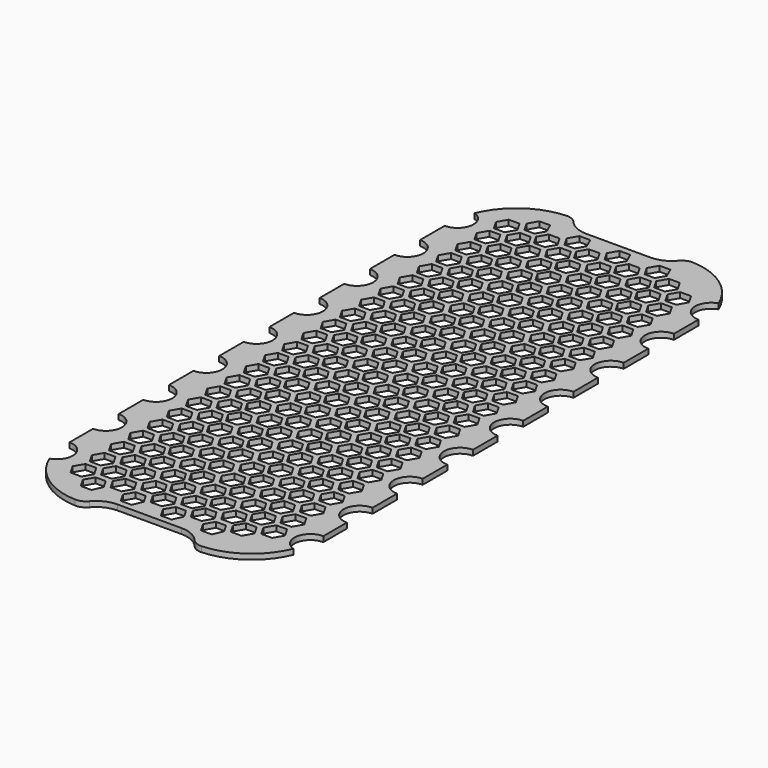
from build123d import *

# Parameters (mm, degrees)
F0_W        = 95
F0_H        = 230
F1_DEPTH    = 2
F2_R        = 25
F3_R        = 6
F3_W        = 41.7297072709
F3_H        = 10
F4_DEPTH    = 10
F5_T1_DEPTH = 2
F6_R        = 5
F8_DEPTH    = 10


# Not quite as in the source:
# - a fillet or chamfer that OpenCascade refuses, or shapes differently, is made with other operations: its cross-section is extruded or revolved along the edge and cut away or added


with BuildPart() as f1:
    # F0 (on Top) → F1 (new body)
    with BuildSketch(Plane.XY):
        Rectangle(F0_W, F0_H)
    extrude(amount=F1_DEPTH)

    # F2
    f2_edges = [f1.edges().sort_by_distance(p)[0] for p in [
        (-47.5, -115, 1),
        (-47.5, 115, 1),
        (47.5, 115, 1),
        (47.5, -115, 1),
    ]]
    fillet(f2_edges, radius=F2_R)

    # F3 (on Top) → F4 (cut)
    with BuildSketch(Plane.XY):
        with Locations((-47.4763996899, 93.75)):
            Circle(F3_R)
        with Locations((47.4763996899, 93.75)):
            Circle(F3_R)
        with Locations((-47.4763996899, -93.75)):
            Circle(F3_R)
        with Locations((47.4763996899, -93.75)):
            Circle(F3_R)
        with Locations((-47.4763996899, 70.25)):
            Circle(F3_R)
        with Locations((-47.4763996899, 46.75)):
            Circle(F3_R)
        with Locations((-47.4763996899, 23.25)):
            Circle(F3_R)
        with Locations((-47.4763996899, -0.25)):
            Circle(F3_R)
        with Locations((-47.4763996899, -23.75)):
            Circle(F3_R)
        with Locations((-47.4763996899, -47.25)):
            Circle(F3_R)
        with Locations((47.4763996899, 70.25)):
            Circle(F3_R)
        with Locations((47.4763996899, 46.75)):
            Circle(F3_R)
        with Locations((47.4763996899, 23.25)):
            Circle(F3_R)
        with Locations((47.4763996899, -0.25)):
            Circle(F3_R)
        with Locations((47.4763996899, -23.75)):
            Circle(F3_R)
        with Locations((47.4763996899, -47.25)):
            Circle(F3_R)
        with Locations((47.4763996899, -70.75)):
            Circle(F3_R)
        with Locations((-47.4763996899, -70.75)):
            Circle(F3_R)
        with Locations((0, -114.6645247936)):
            Rectangle(F3_W, F3_H)
        with Locations((0, 114.6645247936)):
            Rectangle(F3_W, F3_H)
    extrude(amount=F4_DEPTH, mode=Mode.SUBTRACT)

    # F5: fillet of radius 10 on 4 edges, made by hand

    # F5_s2 → F5_t1 (join)
    with BuildSketch(Plane.XY):
        with BuildLine():
            ThreePointArc((-12.0193910444, -109.6645247936), (-17.1844056651, -111.1016617229), (-20.8648536354, -115))
            Line((-20.8648536354, -115), (-20.8648536354, -109.6645247936))
            Line((-20.8648536354, -109.6645247936), (-12.0193910444, -109.6645247936))
        make_face()
        with BuildLine():
            ThreePointArc((20.8648536354, -115), (17.1844056651, -111.1016617229), (12.0193910444, -109.6645247936))
            Line((12.0193910444, -109.6645247936), (20.8648536354, -109.6645247936))
            Line((20.8648536354, -109.6645247936), (20.8648536354, -115))
        make_face()
        with BuildLine():
            ThreePointArc((-20.8648536354, 115), (-17.1844056651, 111.1016617229), (-12.0193910444, 109.6645247936))
            Line((-12.0193910444, 109.6645247936), (-20.8648536354, 109.6645247936))
            Line((-20.8648536354, 109.6645247936), (-20.8648536354, 115))
        make_face()
        with BuildLine():
            ThreePointArc((12.0193910444, 109.6645247936), (17.1844056651, 111.1016617229), (20.8648536354, 115))
            Line((20.8648536354, 115), (20.8648536354, 109.6645247936))
            Line((20.8648536354, 109.6645247936), (12.0193910444, 109.6645247936))
        make_face()
    extrude(amount=F5_T1_DEPTH)

    # F6
    f6_edges = [f1.edges().sort_by_distance(p)[0] for p in [
        (-20.864854, 115, 1),
        (20.864854, 115, 1),
        (-20.864854, -115, 1),
        (20.864854, -115, 1),
    ]]
    fillet(f6_edges, radius=F6_R)

    # F7 (on Top) → F8 (cut)
    with BuildSketch(Plane.XY):
        Polygon((32.4792740578, -91), (30.4585481157, -94.5), (32.4792740578, -98), (36.5207259422, -98), (38.5414518843, -94.5), (36.5207259422, -91), align=None)
        Polygon((32.4725603018, -82.003884784), (30.4585555593, -85.5077566753), (32.4859952575, -89.0038718913), (36.5274396982, -88.996115216), (38.5414444407, -85.4922433247), (36.5140047425, -81.9961281087), align=None)
        Polygon((32.4792740578, -80), (36.5207259422, -80), (38.5414518843, -76.5), (36.5207259422, -73), (32.4792740578, -73), (30.4585481157, -76.5), align=None)
        Polygon((30.4585555593, -67.5077566753), (32.4859952575, -71.0038718913), (36.5274396982, -70.996115216), (38.5414444407, -67.4922433247), (36.5140047425, -63.9961281087), (32.4725603018, -64.003884784), align=None)
        Polygon((32.4792740578, -62), (36.5207259422, -62), (38.5414518843, -58.5), (36.5207259422, -55), (32.4792740578, -55), (30.4585481157, -58.5), align=None)
        Polygon((30.4585555593, -49.5077566753), (32.4859952575, -53.0038718913), (36.5274396982, -52.996115216), (38.5414444407, -49.4922433247), (36.5140047425, -45.9961281087), (32.4725603018, -46.003884784), align=None)
        Polygon((32.4792740578, -44), (36.5207259422, -44), (38.5414518843, -40.5), (36.5207259422, -37), (32.4792740578, -37), (30.4585481157, -40.5), align=None)
        Polygon((30.4585555593, -31.5077566753), (32.4859952575, -35.0038718913), (36.5274396982, -34.996115216), (38.5414444407, -31.4922433247), (36.5140047425, -27.9961281087), (32.4725603018, -28.003884784), align=None)
        Polygon((32.4792740578, -26), (36.5207259422, -26), (38.5414518843, -22.5), (36.5207259422, -19), (32.4792740578, -19), (30.4585481157, -22.5), align=None)
        Polygon((30.4585555593, -13.5077566753), (32.4859952575, -17.0038718913), (36.5274396982, -16.996115216), (38.5414444407, -13.4922433247), (36.5140047425, -9.9961281087), (32.4725603018, -10.003884784), align=None)
        Polygon((32.4792740578, -8), (36.5207259422, -8), (38.5414518843, -4.5), (36.5207259422, -1), (32.4792740578, -1), (30.4585481157, -4.5), align=None)
        Polygon((30.4585555593, 4.4922433247), (32.4859952575, 0.9961281087), (36.5274396982, 1.003884784), (38.5414444407, 4.5077566753), (36.5140047425, 8.0038718913), (32.4725603018, 7.996115216), align=None)
        Polygon((32.4792740578, 10), (36.5207259422, 10), (38.5414518843, 13.5), (36.5207259422, 17), (32.4792740578, 17), (30.4585481157, 13.5), align=None)
        Polygon((30.4585555593, 22.4922433247), (32.4859952575, 18.9961281087), (36.5274396982, 19.003884784), (38.5414444407, 22.5077566753), (36.5140047425, 26.0038718913), (32.4725603018, 25.996115216), align=None)
        Polygon((32.4792740578, 28), (36.5207259422, 28), (38.5414518843, 31.5), (36.5207259422, 35), (32.4792740578, 35), (30.4585481157, 31.5), align=None)
        Polygon((30.4585555593, 40.4922433247), (32.4859952575, 36.9961281087), (36.5274396982, 37.003884784), (38.5414444407, 40.5077566753), (36.5140047425, 44.0038718913), (32.4725603018, 43.996115216), align=None)
        Polygon((32.4792740578, 46), (36.5207259422, 46), (38.5414518843, 49.5), (36.5207259422, 53), (32.4792740578, 53), (30.4585481157, 49.5), align=None)
        Polygon((30.4585555593, 58.4922433247), (32.4859952575, 54.9961281087), (36.5274396982, 55.003884784), (38.5414444407, 58.5077566753), (36.5140047425, 62.0038718913), (32.4725603018, 61.996115216), align=None)
        Polygon((32.4792740578, 64), (36.5207259422, 64), (38.5414518843, 67.5), (36.5207259422, 71), (32.4792740578, 71), (30.4585481157, 67.5), align=None)
        Polygon((30.4585555593, 76.4922433247), (32.4859952575, 72.9961281087), (36.5274396982, 73.003884784), (38.5414444407, 76.5077566753), (36.5140047425, 80.0038718913), (32.4725603018, 79.996115216), align=None)
        Polygon((32.4792740578, 82), (36.5207259422, 82), (38.5414518843, 85.5), (36.5207259422, 89), (32.4792740578, 89), (30.4585481157, 85.5), align=None)
        Polygon((30.4585555593, 94.4922433247), (32.4859952575, 90.9961281087), (36.5274396982, 91.003884784), (38.5414444407, 94.5077566753), (36.5140047425, 98.0038718913), (32.4725603018, 97.996115216), align=None)
        Polygon((28.7264973081, -95.5), (24.6850454238, -95.5), (22.6643194816, -99), (24.6850454238, -102.5), (28.7264973081, -102.5), (30.7472232503, -99), align=None)
        Polygon((28.7264973081, -93.5), (30.7472232503, -90), (28.7264973081, -86.5), (24.6850454238, -86.5), (22.6643194816, -90), (24.6850454238, -93.5), align=None)
        Polygon((28.7264973081, -84.5), (30.7472232503, -81), (28.7264973081, -77.5), (24.6850454238, -77.5), (22.6643194816, -81), (24.6850454238, -84.5), align=None)
        Polygon((28.7264973081, -75.5), (30.7472232503, -72), (28.7264973081, -68.5), (24.6850454238, -68.5), (22.6643194816, -72), (24.6850454238, -75.5), align=None)
        Polygon((28.7264973081, -66.5), (30.7472232503, -63), (28.7264973081, -59.5), (24.6850454238, -59.5), (22.6643194816, -63), (24.6850454238, -66.5), align=None)
        Polygon((28.7264973081, -57.5), (30.7472232503, -54), (28.7264973081, -50.5), (24.6850454238, -50.5), (22.6643194816, -54), (24.6850454238, -57.5), align=None)
        Polygon((28.7264973081, -48.5), (30.7472232503, -45), (28.7264973081, -41.5), (24.6850454238, -41.5), (22.6643194816, -45), (24.6850454238, -48.5), align=None)
        Polygon((28.7264973081, -39.5), (30.7472232503, -36), (28.7264973081, -32.5), (24.6850454238, -32.5), (22.6643194816, -36), (24.6850454238, -39.5), align=None)
        Polygon((28.7264973081, -30.5), (30.7472232503, -27), (28.7264973081, -23.5), (24.6850454238, -23.5), (22.6643194816, -27), (24.6850454238, -30.5), align=None)
        Polygon((28.7264973081, -21.5), (30.7472232503, -18), (28.7264973081, -14.5), (24.6850454238, -14.5), (22.6643194816, -18), (24.6850454238, -21.5), align=None)
        Polygon((28.7264973081, -12.5), (30.7472232503, -9), (28.7264973081, -5.5), (24.6850454238, -5.5), (22.6643194816, -9), (24.6850454238, -12.5), align=None)
        Polygon((28.7264973081, -3.5), (30.7472232503, 0), (28.7264973081, 3.5), (24.6850454238, 3.5), (22.6643194816, 0), (24.6850454238, -3.5), align=None)
        Polygon((28.7264973081, 5.5), (30.7472232503, 9), (28.7264973081, 12.5), (24.6850454238, 12.5), (22.6643194816, 9), (24.6850454238, 5.5), align=None)
        Polygon((28.7264973081, 14.5), (30.7472232503, 18), (28.7264973081, 21.5), (24.6850454238, 21.5), (22.6643194816, 18), (24.6850454238, 14.5), align=None)
        Polygon((28.7264973081, 23.5), (30.7472232503, 27), (28.7264973081, 30.5), (24.6850454238, 30.5), (22.6643194816, 27), (24.6850454238, 23.5), align=None)
        Polygon((28.7264973081, 32.5), (30.7472232503, 36), (28.7264973081, 39.5), (24.6850454238, 39.5), (22.6643194816, 36), (24.6850454238, 32.5), align=None)
        Polygon((28.7264973081, 41.5), (30.7472232503, 45), (28.7264973081, 48.5), (24.6850454238, 48.5), (22.6643194816, 45), (24.6850454238, 41.5), align=None)
        Polygon((28.7264973081, 50.5), (30.7472232503, 54), (28.7264973081, 57.5), (24.6850454238, 57.5), (22.6643194816, 54), (24.6850454238, 50.5), align=None)
        Polygon((28.7264973081, 59.5), (30.7472232503, 63), (28.7264973081, 66.5), (24.6850454238, 66.5), (22.6643194816, 63), (24.6850454238, 59.5), align=None)
        Polygon((28.7264973081, 68.5), (30.7472232503, 72), (28.7264973081, 75.5), (24.6850454238, 75.5), (22.6643194816, 72), (24.6850454238, 68.5), align=None)
        Polygon((28.7264973081, 77.5), (30.7472232503, 81), (28.7264973081, 84.5), (24.6850454238, 84.5), (22.6643194816, 81), (24.6850454238, 77.5), align=None)
        Polygon((28.7264973081, 86.5), (30.7472232503, 90), (28.7264973081, 93.5), (24.6850454238, 93.5), (22.6643194816, 90), (24.6850454238, 86.5), align=None)
        Polygon((28.7264973081, 95.5), (30.7472232503, 99), (28.7264973081, 102.5), (24.6850454238, 102.5), (22.6643194816, 99), (24.6850454238, 95.5), align=None)
        Polygon((21.5140047425, -45.9961281087), (17.4725603018, -46.003884784), (15.4585555593, -49.5077566753), (17.4859952575, -53.0038718913), (21.5274396982, -52.996115216), (23.5414444407, -49.4922433247), align=None)
        Polygon((21.5207259422, -55), (17.4792740578, -55), (15.4585481157, -58.5), (17.4792740578, -62), (21.5207259422, -62), (23.5414518843, -58.5), align=None)
        Polygon((13.7264973081, -41.5), (9.6850454238, -41.5), (7.6643194816, -45), (9.6850454238, -48.5), (13.7264973081, -48.5), (15.7472232503, -45), align=None)
        Polygon((13.7264973081, -32.5), (9.6850454238, -32.5), (7.6643194816, -36), (9.6850454238, -39.5), (13.7264973081, -39.5), (15.7472232503, -36), align=None)
        Polygon((13.7264973081, -59.5), (9.6850454238, -59.5), (7.6643194816, -63), (9.6850454238, -66.5), (13.7264973081, -66.5), (15.7472232503, -63), align=None)
        Polygon((13.7264973081, -77.5), (9.6850454238, -77.5), (7.6643194816, -81), (9.6850454238, -84.5), (13.7264973081, -84.5), (15.7472232503, -81), align=None)
        Polygon((21.5207259422, -73), (17.4792740578, -73), (15.4585481157, -76.5), (17.4792740578, -80), (21.5207259422, -80), (23.5414518843, -76.5), align=None)
        Polygon((21.5207259422, -37), (17.4792740578, -37), (15.4585481157, -40.5), (17.4792740578, -44), (21.5207259422, -44), (23.5414518843, -40.5), align=None)
        Polygon((13.7264973081, -86.5), (9.6850454238, -86.5), (7.6643194816, -90), (9.6850454238, -93.5), (13.7264973081, -93.5), (15.7472232503, -90), align=None)
        Polygon((13.7264973081, -50.5), (9.6850454238, -50.5), (7.6643194816, -54), (9.6850454238, -57.5), (13.7264973081, -57.5), (15.7472232503, -54), align=None)
        Polygon((21.5140047425, -63.9961281087), (17.4725603018, -64.003884784), (15.4585555593, -67.5077566753), (17.4859952575, -71.0038718913), (21.5274396982, -70.996115216), (23.5414444407, -67.4922433247), align=None)
        Polygon((13.7264973081, -68.5), (9.6850454238, -68.5), (7.6643194816, -72), (9.6850454238, -75.5), (13.7264973081, -75.5), (15.7472232503, -72), align=None)
        Polygon((21.5140047425, -27.9961281087), (17.4725603018, -28.003884784), (15.4585555593, -31.5077566753), (17.4859952575, -35.0038718913), (21.5274396982, -34.996115216), (23.5414444407, -31.4922433247), align=None)
        Polygon((13.7264973081, -23.5), (9.6850454238, -23.5), (7.6643194816, -27), (9.6850454238, -30.5), (13.7264973081, -30.5), (15.7472232503, -27), align=None)
        Polygon((21.5207259422, -91), (17.4792740578, -91), (15.4585481157, -94.5), (17.4792740578, -98), (21.5207259422, -98), (23.5414518843, -94.5), align=None)
        Polygon((23.5414444407, -13.4922433247), (21.5140047425, -9.9961281087), (17.4725603018, -10.003884784), (15.4585555593, -13.5077566753), (17.4859952575, -17.0038718913), (21.5274396982, -16.996115216), align=None)
        Polygon((9.6850454238, -12.5), (13.7264973081, -12.5), (15.7472232503, -9), (13.7264973081, -5.5), (9.6850454238, -5.5), (7.6643194816, -9), align=None)
        Polygon((17.4792740578, 28), (21.5207259422, 28), (23.5414518843, 31.5), (21.5207259422, 35), (17.4792740578, 35), (15.4585481157, 31.5), align=None)
        Polygon((17.4859952575, -89.0038718913), (21.5274396982, -88.996115216), (23.5414444407, -85.4922433247), (21.5140047425, -81.9961281087), (17.4725603018, -82.003884784), (15.4585555593, -85.5077566753), align=None)
        Polygon((9.6850454238, 14.5), (13.7264973081, 14.5), (15.7472232503, 18), (13.7264973081, 21.5), (9.6850454238, 21.5), (7.6643194816, 18), align=None)
        Polygon((17.4792740578, -8), (21.5207259422, -8), (23.5414518843, -4.5), (21.5207259422, -1), (17.4792740578, -1), (15.4585481157, -4.5), align=None)
        Polygon((13.7264973081, 30.5), (9.6850454238, 30.5), (7.6643194816, 27), (9.6850454238, 23.5), (13.7264973081, 23.5), (15.7472232503, 27), align=None)
        Polygon((13.7264973081, -14.5), (9.6850454238, -14.5), (7.6643194816, -18), (9.6850454238, -21.5), (13.7264973081, -21.5), (15.7472232503, -18), align=None)
        Polygon((13.7264973081, -95.5), (9.6850454238, -95.5), (7.6643194816, -99), (9.6850454238, -102.5), (13.7264973081, -102.5), (15.7472232503, -99), align=None)
        Polygon((9.6850454238, 77.5), (13.7264973081, 77.5), (15.7472232503, 81), (13.7264973081, 84.5), (9.6850454238, 84.5), (7.6643194816, 81), align=None)
        Polygon((21.5207259422, 17), (17.4792740578, 17), (15.4585481157, 13.5), (17.4792740578, 10), (21.5207259422, 10), (23.5414518843, 13.5), align=None)
        Polygon((9.6850454238, 32.5), (13.7264973081, 32.5), (15.7472232503, 36), (13.7264973081, 39.5), (9.6850454238, 39.5), (7.6643194816, 36), align=None)
        Polygon((9.6850454238, 50.5), (13.7264973081, 50.5), (15.7472232503, 54), (13.7264973081, 57.5), (9.6850454238, 57.5), (7.6643194816, 54), align=None)
        Polygon((21.5207259422, 71), (17.4792740578, 71), (15.4585481157, 67.5), (17.4792740578, 64), (21.5207259422, 64), (23.5414518843, 67.5), align=None)
        Polygon((21.5140047425, 80.0038718913), (17.4725603018, 79.996115216), (15.4585555593, 76.4922433247), (17.4859952575, 72.9961281087), (21.5274396982, 73.003884784), (23.5414444407, 76.5077566753), align=None)
        Polygon((17.4792740578, 46), (21.5207259422, 46), (23.5414518843, 49.5), (21.5207259422, 53), (17.4792740578, 53), (15.4585481157, 49.5), align=None)
        Polygon((17.4792740578, 82), (21.5207259422, 82), (23.5414518843, 85.5), (21.5207259422, 89), (17.4792740578, 89), (15.4585481157, 85.5), align=None)
        Polygon((17.4792740578, -26), (21.5207259422, -26), (23.5414518843, -22.5), (21.5207259422, -19), (17.4792740578, -19), (15.4585481157, -22.5), align=None)
        Polygon((17.4859952575, 36.9961281087), (21.5274396982, 37.003884784), (23.5414444407, 40.5077566753), (21.5140047425, 44.0038718913), (17.4725603018, 43.996115216), (15.4585555593, 40.4922433247), align=None)
        Polygon((17.4859952575, 90.9961281087), (21.5274396982, 91.003884784), (23.5414444407, 94.5077566753), (21.5140047425, 98.0038718913), (17.4725603018, 97.996115216), (15.4585555593, 94.4922433247), align=None)
        Polygon((9.6850454238, 41.5), (13.7264973081, 41.5), (15.7472232503, 45), (13.7264973081, 48.5), (9.6850454238, 48.5), (7.6643194816, 45), align=None)
        Polygon((9.6850454238, 86.5), (13.7264973081, 86.5), (15.7472232503, 90), (13.7264973081, 93.5), (9.6850454238, 93.5), (7.6643194816, 90), align=None)
        Polygon((13.7264973081, 75.5), (9.6850454238, 75.5), (7.6643194816, 72), (9.6850454238, 68.5), (13.7264973081, 68.5), (15.7472232503, 72), align=None)
        Polygon((17.4859952575, 18.9961281087), (21.5274396982, 19.003884784), (23.5414444407, 22.5077566753), (21.5140047425, 26.0038718913), (17.4725603018, 25.996115216), (15.4585555593, 22.4922433247), align=None)
        Polygon((9.6850454238, 59.5), (13.7264973081, 59.5), (15.7472232503, 63), (13.7264973081, 66.5), (9.6850454238, 66.5), (7.6643194816, 63), align=None)
        Polygon((17.4859952575, 0.9961281087), (21.5274396982, 1.003884784), (23.5414444407, 4.5077566753), (21.5140047425, 8.0038718913), (17.4725603018, 7.996115216), (15.4585555593, 4.4922433247), align=None)
        Polygon((9.6850454238, -3.5), (13.7264973081, -3.5), (15.7472232503, 0), (13.7264973081, 3.5), (9.6850454238, 3.5), (7.6643194816, 0), align=None)
        Polygon((21.5140047425, 62.0038718913), (17.4725603018, 61.996115216), (15.4585555593, 58.4922433247), (17.4859952575, 54.9961281087), (21.5274396982, 55.003884784), (23.5414444407, 58.5077566753), align=None)
        Polygon((13.7264973081, 102.5), (9.6850454238, 102.5), (7.6643194816, 99), (9.6850454238, 95.5), (13.7264973081, 95.5), (15.7472232503, 99), align=None)
        Polygon((13.7264973081, 12.5), (9.6850454238, 12.5), (7.6643194816, 9), (9.6850454238, 5.5), (13.7264973081, 5.5), (15.7472232503, 9), align=None)
        Polygon((6.5140047425, -45.9961281087), (2.4725603018, -46.003884784), (0.4585555593, -49.5077566753), (2.4859952575, -53.0038718913), (6.5274396982, -52.996115216), (8.5414444407, -49.4922433247), align=None)
        Polygon((6.5207259422, -55), (2.4792740578, -55), (0.4585481157, -58.5), (2.4792740578, -62), (6.5207259422, -62), (8.5414518843, -58.5), align=None)
        Polygon((-1.2735026919, -41.5), (-5.3149545762, -41.5), (-7.3356805184, -45), (-5.3149545762, -48.5), (-1.2735026919, -48.5), (0.7472232503, -45), align=None)
        Polygon((-1.2735026919, -32.5), (-5.3149545762, -32.5), (-7.3356805184, -36), (-5.3149545762, -39.5), (-1.2735026919, -39.5), (0.7472232503, -36), align=None)
        Polygon((-1.2735026919, -59.5), (-5.3149545762, -59.5), (-7.3356805184, -63), (-5.3149545762, -66.5), (-1.2735026919, -66.5), (0.7472232503, -63), align=None)
        Polygon((-1.2735026919, -77.5), (-5.3149545762, -77.5), (-7.3356805184, -81), (-5.3149545762, -84.5), (-1.2735026919, -84.5), (0.7472232503, -81), align=None)
        Polygon((6.5207259422, -73), (2.4792740578, -73), (0.4585481157, -76.5), (2.4792740578, -80), (6.5207259422, -80), (8.5414518843, -76.5), align=None)
        Polygon((6.5207259422, -37), (2.4792740578, -37), (0.4585481157, -40.5), (2.4792740578, -44), (6.5207259422, -44), (8.5414518843, -40.5), align=None)
        Polygon((-1.2735026919, -86.5), (-5.3149545762, -86.5), (-7.3356805184, -90), (-5.3149545762, -93.5), (-1.2735026919, -93.5), (0.7472232503, -90), align=None)
        Polygon((-1.2735026919, -50.5), (-5.3149545762, -50.5), (-7.3356805184, -54), (-5.3149545762, -57.5), (-1.2735026919, -57.5), (0.7472232503, -54), align=None)
        Polygon((6.5140047425, -63.9961281087), (2.4725603018, -64.003884784), (0.4585555593, -67.5077566753), (2.4859952575, -71.0038718913), (6.5274396982, -70.996115216), (8.5414444407, -67.4922433247), align=None)
        Polygon((-1.2735026919, -68.5), (-5.3149545762, -68.5), (-7.3356805184, -72), (-5.3149545762, -75.5), (-1.2735026919, -75.5), (0.7472232503, -72), align=None)
        Polygon((6.5140047425, -27.9961281087), (2.4725603018, -28.003884784), (0.4585555593, -31.5077566753), (2.4859952575, -35.0038718913), (6.5274396982, -34.996115216), (8.5414444407, -31.4922433247), align=None)
        Polygon((-1.2735026919, -23.5), (-5.3149545762, -23.5), (-7.3356805184, -27), (-5.3149545762, -30.5), (-1.2735026919, -30.5), (0.7472232503, -27), align=None)
        Polygon((6.5207259422, -91), (2.4792740578, -91), (0.4585481157, -94.5), (2.4792740578, -98), (6.5207259422, -98), (8.5414518843, -94.5), align=None)
        Polygon((8.5414444407, -13.4922433247), (6.5140047425, -9.9961281087), (2.4725603018, -10.003884784), (0.4585555593, -13.5077566753), (2.4859952575, -17.0038718913), (6.5274396982, -16.996115216), align=None)
        Polygon((-5.3149545762, -12.5), (-1.2735026919, -12.5), (0.7472232503, -9), (-1.2735026919, -5.5), (-5.3149545762, -5.5), (-7.3356805184, -9), align=None)
        Polygon((2.4792740578, 28), (6.5207259422, 28), (8.5414518843, 31.5), (6.5207259422, 35), (2.4792740578, 35), (0.4585481157, 31.5), align=None)
        Polygon((2.4859952575, -89.0038718913), (6.5274396982, -88.996115216), (8.5414444407, -85.4922433247), (6.5140047425, -81.9961281087), (2.4725603018, -82.003884784), (0.4585555593, -85.5077566753), align=None)
        Polygon((-5.3149545762, 14.5), (-1.2735026919, 14.5), (0.7472232503, 18), (-1.2735026919, 21.5), (-5.3149545762, 21.5), (-7.3356805184, 18), align=None)
        Polygon((2.4792740578, -8), (6.5207259422, -8), (8.5414518843, -4.5), (6.5207259422, -1), (2.4792740578, -1), (0.4585481157, -4.5), align=None)
        Polygon((-1.2735026919, 30.5), (-5.3149545762, 30.5), (-7.3356805184, 27), (-5.3149545762, 23.5), (-1.2735026919, 23.5), (0.7472232503, 27), align=None)
        Polygon((-1.2735026919, -14.5), (-5.3149545762, -14.5), (-7.3356805184, -18), (-5.3149545762, -21.5), (-1.2735026919, -21.5), (0.7472232503, -18), align=None)
        Polygon((-1.2735026919, -95.5), (-5.3149545762, -95.5), (-7.3356805184, -99), (-5.3149545762, -102.5), (-1.2735026919, -102.5), (0.7472232503, -99), align=None)
        Polygon((-5.3149545762, 77.5), (-1.2735026919, 77.5), (0.7472232503, 81), (-1.2735026919, 84.5), (-5.3149545762, 84.5), (-7.3356805184, 81), align=None)
        Polygon((6.5207259422, 17), (2.4792740578, 17), (0.4585481157, 13.5), (2.4792740578, 10), (6.5207259422, 10), (8.5414518843, 13.5), align=None)
        Polygon((-5.3149545762, 32.5), (-1.2735026919, 32.5), (0.7472232503, 36), (-1.2735026919, 39.5), (-5.3149545762, 39.5), (-7.3356805184, 36), align=None)
        Polygon((-5.3149545762, 50.5), (-1.2735026919, 50.5), (0.7472232503, 54), (-1.2735026919, 57.5), (-5.3149545762, 57.5), (-7.3356805184, 54), align=None)
        Polygon((6.5207259422, 71), (2.4792740578, 71), (0.4585481157, 67.5), (2.4792740578, 64), (6.5207259422, 64), (8.5414518843, 67.5), align=None)
        Polygon((6.5140047425, 80.0038718913), (2.4725603018, 79.996115216), (0.4585555593, 76.4922433247), (2.4859952575, 72.9961281087), (6.5274396982, 73.003884784), (8.5414444407, 76.5077566753), align=None)
        Polygon((2.4792740578, 46), (6.5207259422, 46), (8.5414518843, 49.5), (6.5207259422, 53), (2.4792740578, 53), (0.4585481157, 49.5), align=None)
        Polygon((2.4792740578, 82), (6.5207259422, 82), (8.5414518843, 85.5), (6.5207259422, 89), (2.4792740578, 89), (0.4585481157, 85.5), align=None)
        Polygon((2.4792740578, -26), (6.5207259422, -26), (8.5414518843, -22.5), (6.5207259422, -19), (2.4792740578, -19), (0.4585481157, -22.5), align=None)
        Polygon((2.4859952575, 36.9961281087), (6.5274396982, 37.003884784), (8.5414444407, 40.5077566753), (6.5140047425, 44.0038718913), (2.4725603018, 43.996115216), (0.4585555593, 40.4922433247), align=None)
        Polygon((2.4859952575, 90.9961281087), (6.5274396982, 91.003884784), (8.5414444407, 94.5077566753), (6.5140047425, 98.0038718913), (2.4725603018, 97.996115216), (0.4585555593, 94.4922433247), align=None)
        Polygon((-5.3149545762, 41.5), (-1.2735026919, 41.5), (0.7472232503, 45), (-1.2735026919, 48.5), (-5.3149545762, 48.5), (-7.3356805184, 45), align=None)
        Polygon((-5.3149545762, 86.5), (-1.2735026919, 86.5), (0.7472232503, 90), (-1.2735026919, 93.5), (-5.3149545762, 93.5), (-7.3356805184, 90), align=None)
        Polygon((-1.2735026919, 75.5), (-5.3149545762, 75.5), (-7.3356805184, 72), (-5.3149545762, 68.5), (-1.2735026919, 68.5), (0.7472232503, 72), align=None)
        Polygon((2.4859952575, 18.9961281087), (6.5274396982, 19.003884784), (8.5414444407, 22.5077566753), (6.5140047425, 26.0038718913), (2.4725603018, 25.996115216), (0.4585555593, 22.4922433247), align=None)
        Polygon((-5.3149545762, 59.5), (-1.2735026919, 59.5), (0.7472232503, 63), (-1.2735026919, 66.5), (-5.3149545762, 66.5), (-7.3356805184, 63), align=None)
        Polygon((2.4859952575, 0.9961281087), (6.5274396982, 1.003884784), (8.5414444407, 4.5077566753), (6.5140047425, 8.0038718913), (2.4725603018, 7.996115216), (0.4585555593, 4.4922433247), align=None)
        Polygon((-5.3149545762, -3.5), (-1.2735026919, -3.5), (0.7472232503, 0), (-1.2735026919, 3.5), (-5.3149545762, 3.5), (-7.3356805184, 0), align=None)
        Polygon((6.5140047425, 62.0038718913), (2.4725603018, 61.996115216), (0.4585555593, 58.4922433247), (2.4859952575, 54.9961281087), (6.5274396982, 55.003884784), (8.5414444407, 58.5077566753), align=None)
        Polygon((-1.2735026919, 102.5), (-5.3149545762, 102.5), (-7.3356805184, 99), (-5.3149545762, 95.5), (-1.2735026919, 95.5), (0.7472232503, 99), align=None)
        Polygon((-1.2735026919, 12.5), (-5.3149545762, 12.5), (-7.3356805184, 9), (-5.3149545762, 5.5), (-1.2735026919, 5.5), (0.7472232503, 9), align=None)
        Polygon((-8.4859952575, -45.9961281087), (-12.5274396982, -46.003884784), (-14.5414444407, -49.5077566753), (-12.5140047425, -53.0038718913), (-8.4725603018, -52.996115216), (-6.4585555593, -49.4922433247), align=None)
        Polygon((-8.4792740578, -55), (-12.5207259422, -55), (-14.5414518843, -58.5), (-12.5207259422, -62), (-8.4792740578, -62), (-6.4585481157, -58.5), align=None)
        Polygon((-16.2735026919, -41.5), (-20.3149545762, -41.5), (-22.3356805184, -45), (-20.3149545762, -48.5), (-16.2735026919, -48.5), (-14.2527767497, -45), align=None)
        Polygon((-16.2735026919, -32.5), (-20.3149545762, -32.5), (-22.3356805184, -36), (-20.3149545762, -39.5), (-16.2735026919, -39.5), (-14.2527767497, -36), align=None)
        Polygon((-16.2735026919, -59.5), (-20.3149545762, -59.5), (-22.3356805184, -63), (-20.3149545762, -66.5), (-16.2735026919, -66.5), (-14.2527767497, -63), align=None)
        Polygon((-16.2735026919, -77.5), (-20.3149545762, -77.5), (-22.3356805184, -81), (-20.3149545762, -84.5), (-16.2735026919, -84.5), (-14.2527767497, -81), align=None)
        Polygon((-8.4792740578, -73), (-12.5207259422, -73), (-14.5414518843, -76.5), (-12.5207259422, -80), (-8.4792740578, -80), (-6.4585481157, -76.5), align=None)
        Polygon((-8.4792740578, -37), (-12.5207259422, -37), (-14.5414518843, -40.5), (-12.5207259422, -44), (-8.4792740578, -44), (-6.4585481157, -40.5), align=None)
        Polygon((-16.2735026919, -86.5), (-20.3149545762, -86.5), (-22.3356805184, -90), (-20.3149545762, -93.5), (-16.2735026919, -93.5), (-14.2527767497, -90), align=None)
        Polygon((-16.2735026919, -50.5), (-20.3149545762, -50.5), (-22.3356805184, -54), (-20.3149545762, -57.5), (-16.2735026919, -57.5), (-14.2527767497, -54), align=None)
        Polygon((-8.4859952575, -63.9961281087), (-12.5274396982, -64.003884784), (-14.5414444407, -67.5077566753), (-12.5140047425, -71.0038718913), (-8.4725603018, -70.996115216), (-6.4585555593, -67.4922433247), align=None)
        Polygon((-16.2735026919, -68.5), (-20.3149545762, -68.5), (-22.3356805184, -72), (-20.3149545762, -75.5), (-16.2735026919, -75.5), (-14.2527767497, -72), align=None)
        Polygon((-8.4859952575, -27.9961281087), (-12.5274396982, -28.003884784), (-14.5414444407, -31.5077566753), (-12.5140047425, -35.0038718913), (-8.4725603018, -34.996115216), (-6.4585555593, -31.4922433247), align=None)
        Polygon((-16.2735026919, -23.5), (-20.3149545762, -23.5), (-22.3356805184, -27), (-20.3149545762, -30.5), (-16.2735026919, -30.5), (-14.2527767497, -27), align=None)
        Polygon((-8.4792740578, -91), (-12.5207259422, -91), (-14.5414518843, -94.5), (-12.5207259422, -98), (-8.4792740578, -98), (-6.4585481157, -94.5), align=None)
        Polygon((-6.4585555593, -13.4922433247), (-8.4859952575, -9.9961281087), (-12.5274396982, -10.003884784), (-14.5414444407, -13.5077566753), (-12.5140047425, -17.0038718913), (-8.4725603018, -16.996115216), align=None)
        Polygon((-20.3149545762, -12.5), (-16.2735026919, -12.5), (-14.2527767497, -9), (-16.2735026919, -5.5), (-20.3149545762, -5.5), (-22.3356805184, -9), align=None)
        Polygon((-12.5207259422, 28), (-8.4792740578, 28), (-6.4585481157, 31.5), (-8.4792740578, 35), (-12.5207259422, 35), (-14.5414518843, 31.5), align=None)
        Polygon((-12.5140047425, -89.0038718913), (-8.4725603018, -88.996115216), (-6.4585555593, -85.4922433247), (-8.4859952575, -81.9961281087), (-12.5274396982, -82.003884784), (-14.5414444407, -85.5077566753), align=None)
        Polygon((-20.3149545762, 14.5), (-16.2735026919, 14.5), (-14.2527767497, 18), (-16.2735026919, 21.5), (-20.3149545762, 21.5), (-22.3356805184, 18), align=None)
        Polygon((-12.5207259422, -8), (-8.4792740578, -8), (-6.4585481157, -4.5), (-8.4792740578, -1), (-12.5207259422, -1), (-14.5414518843, -4.5), align=None)
        Polygon((-16.2735026919, 30.5), (-20.3149545762, 30.5), (-22.3356805184, 27), (-20.3149545762, 23.5), (-16.2735026919, 23.5), (-14.2527767497, 27), align=None)
        Polygon((-16.2735026919, -14.5), (-20.3149545762, -14.5), (-22.3356805184, -18), (-20.3149545762, -21.5), (-16.2735026919, -21.5), (-14.2527767497, -18), align=None)
        Polygon((-16.2735026919, -95.5), (-20.3149545762, -95.5), (-22.3356805184, -99), (-20.3149545762, -102.5), (-16.2735026919, -102.5), (-14.2527767497, -99), align=None)
        Polygon((-20.3149545762, 77.5), (-16.2735026919, 77.5), (-14.2527767497, 81), (-16.2735026919, 84.5), (-20.3149545762, 84.5), (-22.3356805184, 81), align=None)
        Polygon((-8.4792740578, 17), (-12.5207259422, 17), (-14.5414518843, 13.5), (-12.5207259422, 10), (-8.4792740578, 10), (-6.4585481157, 13.5), align=None)
        Polygon((-20.3149545762, 32.5), (-16.2735026919, 32.5), (-14.2527767497, 36), (-16.2735026919, 39.5), (-20.3149545762, 39.5), (-22.3356805184, 36), align=None)
        Polygon((-20.3149545762, 50.5), (-16.2735026919, 50.5), (-14.2527767497, 54), (-16.2735026919, 57.5), (-20.3149545762, 57.5), (-22.3356805184, 54), align=None)
        Polygon((-8.4792740578, 71), (-12.5207259422, 71), (-14.5414518843, 67.5), (-12.5207259422, 64), (-8.4792740578, 64), (-6.4585481157, 67.5), align=None)
        Polygon((-8.4859952575, 80.0038718913), (-12.5274396982, 79.996115216), (-14.5414444407, 76.4922433247), (-12.5140047425, 72.9961281087), (-8.4725603018, 73.003884784), (-6.4585555593, 76.5077566753), align=None)
        Polygon((-12.5207259422, 46), (-8.4792740578, 46), (-6.4585481157, 49.5), (-8.4792740578, 53), (-12.5207259422, 53), (-14.5414518843, 49.5), align=None)
        Polygon((-12.5207259422, 82), (-8.4792740578, 82), (-6.4585481157, 85.5), (-8.4792740578, 89), (-12.5207259422, 89), (-14.5414518843, 85.5), align=None)
        Polygon((-12.5207259422, -26), (-8.4792740578, -26), (-6.4585481157, -22.5), (-8.4792740578, -19), (-12.5207259422, -19), (-14.5414518843, -22.5), align=None)
        Polygon((-12.5140047425, 36.9961281087), (-8.4725603018, 37.003884784), (-6.4585555593, 40.5077566753), (-8.4859952575, 44.0038718913), (-12.5274396982, 43.996115216), (-14.5414444407, 40.4922433247), align=None)
        Polygon((-12.5140047425, 90.9961281087), (-8.4725603018, 91.003884784), (-6.4585555593, 94.5077566753), (-8.4859952575, 98.0038718913), (-12.5274396982, 97.996115216), (-14.5414444407, 94.4922433247), align=None)
        Polygon((-20.3149545762, 41.5), (-16.2735026919, 41.5), (-14.2527767497, 45), (-16.2735026919, 48.5), (-20.3149545762, 48.5), (-22.3356805184, 45), align=None)
        Polygon((-20.3149545762, 86.5), (-16.2735026919, 86.5), (-14.2527767497, 90), (-16.2735026919, 93.5), (-20.3149545762, 93.5), (-22.3356805184, 90), align=None)
        Polygon((-16.2735026919, 75.5), (-20.3149545762, 75.5), (-22.3356805184, 72), (-20.3149545762, 68.5), (-16.2735026919, 68.5), (-14.2527767497, 72), align=None)
        Polygon((-12.5140047425, 18.9961281087), (-8.4725603018, 19.003884784), (-6.4585555593, 22.5077566753), (-8.4859952575, 26.0038718913), (-12.5274396982, 25.996115216), (-14.5414444407, 22.4922433247), align=None)
        Polygon((-20.3149545762, 59.5), (-16.2735026919, 59.5), (-14.2527767497, 63), (-16.2735026919, 66.5), (-20.3149545762, 66.5), (-22.3356805184, 63), align=None)
        Polygon((-12.5140047425, 0.9961281087), (-8.4725603018, 1.003884784), (-6.4585555593, 4.5077566753), (-8.4859952575, 8.0038718913), (-12.5274396982, 7.996115216), (-14.5414444407, 4.4922433247), align=None)
        Polygon((-20.3149545762, -3.5), (-16.2735026919, -3.5), (-14.2527767497, 0), (-16.2735026919, 3.5), (-20.3149545762, 3.5), (-22.3356805184, 0), align=None)
        Polygon((-8.4859952575, 62.0038718913), (-12.5274396982, 61.996115216), (-14.5414444407, 58.4922433247), (-12.5140047425, 54.9961281087), (-8.4725603018, 55.003884784), (-6.4585555593, 58.5077566753), align=None)
        Polygon((-16.2735026919, 102.5), (-20.3149545762, 102.5), (-22.3356805184, 99), (-20.3149545762, 95.5), (-16.2735026919, 95.5), (-14.2527767497, 99), align=None)
        Polygon((-16.2735026919, 12.5), (-20.3149545762, 12.5), (-22.3356805184, 9), (-20.3149545762, 5.5), (-16.2735026919, 5.5), (-14.2527767497, 9), align=None)
        Polygon((-23.4859952575, -45.9961281087), (-27.5274396982, -46.003884784), (-29.5414444407, -49.5077566753), (-27.5140047425, -53.0038718913), (-23.4725603018, -52.996115216), (-21.4585555593, -49.4922433247), align=None)
        Polygon((-23.4792740578, -55), (-27.5207259422, -55), (-29.5414518843, -58.5), (-27.5207259422, -62), (-23.4792740578, -62), (-21.4585481157, -58.5), align=None)
        Polygon((-31.2735026919, -41.5), (-35.3149545762, -41.5), (-37.3356805184, -45), (-35.3149545762, -48.5), (-31.2735026919, -48.5), (-29.2527767497, -45), align=None)
        Polygon((-31.2735026919, -32.5), (-35.3149545762, -32.5), (-37.3356805184, -36), (-35.3149545762, -39.5), (-31.2735026919, -39.5), (-29.2527767497, -36), align=None)
        Polygon((-31.2735026919, -59.5), (-35.3149545762, -59.5), (-37.3356805184, -63), (-35.3149545762, -66.5), (-31.2735026919, -66.5), (-29.2527767497, -63), align=None)
        Polygon((-31.2735026919, -77.5), (-35.3149545762, -77.5), (-37.3356805184, -81), (-35.3149545762, -84.5), (-31.2735026919, -84.5), (-29.2527767497, -81), align=None)
        Polygon((-23.4792740578, -73), (-27.5207259422, -73), (-29.5414518843, -76.5), (-27.5207259422, -80), (-23.4792740578, -80), (-21.4585481157, -76.5), align=None)
        Polygon((-23.4792740578, -37), (-27.5207259422, -37), (-29.5414518843, -40.5), (-27.5207259422, -44), (-23.4792740578, -44), (-21.4585481157, -40.5), align=None)
        Polygon((-31.2735026919, -86.5), (-35.3149545762, -86.5), (-37.3356805184, -90), (-35.3149545762, -93.5), (-31.2735026919, -93.5), (-29.2527767497, -90), align=None)
        Polygon((-31.2735026919, -50.5), (-35.3149545762, -50.5), (-37.3356805184, -54), (-35.3149545762, -57.5), (-31.2735026919, -57.5), (-29.2527767497, -54), align=None)
        Polygon((-23.4859952575, -63.9961281087), (-27.5274396982, -64.003884784), (-29.5414444407, -67.5077566753), (-27.5140047425, -71.0038718913), (-23.4725603018, -70.996115216), (-21.4585555593, -67.4922433247), align=None)
        Polygon((-31.2735026919, -68.5), (-35.3149545762, -68.5), (-37.3356805184, -72), (-35.3149545762, -75.5), (-31.2735026919, -75.5), (-29.2527767497, -72), align=None)
        Polygon((-23.4859952575, -27.9961281087), (-27.5274396982, -28.003884784), (-29.5414444407, -31.5077566753), (-27.5140047425, -35.0038718913), (-23.4725603018, -34.996115216), (-21.4585555593, -31.4922433247), align=None)
        Polygon((-31.2735026919, -23.5), (-35.3149545762, -23.5), (-37.3356805184, -27), (-35.3149545762, -30.5), (-31.2735026919, -30.5), (-29.2527767497, -27), align=None)
        Polygon((-23.4792740578, -91), (-27.5207259422, -91), (-29.5414518843, -94.5), (-27.5207259422, -98), (-23.4792740578, -98), (-21.4585481157, -94.5), align=None)
        Polygon((-21.4585555593, -13.4922433247), (-23.4859952575, -9.9961281087), (-27.5274396982, -10.003884784), (-29.5414444407, -13.5077566753), (-27.5140047425, -17.0038718913), (-23.4725603018, -16.996115216), align=None)
        Polygon((-35.3149545762, -12.5), (-31.2735026919, -12.5), (-29.2527767497, -9), (-31.2735026919, -5.5), (-35.3149545762, -5.5), (-37.3356805184, -9), align=None)
        Polygon((-27.5207259422, 28), (-23.4792740578, 28), (-21.4585481157, 31.5), (-23.4792740578, 35), (-27.5207259422, 35), (-29.5414518843, 31.5), align=None)
        Polygon((-27.5140047425, -89.0038718913), (-23.4725603018, -88.996115216), (-21.4585555593, -85.4922433247), (-23.4859952575, -81.9961281087), (-27.5274396982, -82.003884784), (-29.5414444407, -85.5077566753), align=None)
        Polygon((-35.3149545762, 14.5), (-31.2735026919, 14.5), (-29.2527767497, 18), (-31.2735026919, 21.5), (-35.3149545762, 21.5), (-37.3356805184, 18), align=None)
        Polygon((-27.5207259422, -8), (-23.4792740578, -8), (-21.4585481157, -4.5), (-23.4792740578, -1), (-27.5207259422, -1), (-29.5414518843, -4.5), align=None)
        Polygon((-31.2735026919, 30.5), (-35.3149545762, 30.5), (-37.3356805184, 27), (-35.3149545762, 23.5), (-31.2735026919, 23.5), (-29.2527767497, 27), align=None)
        Polygon((-31.2735026919, -14.5), (-35.3149545762, -14.5), (-37.3356805184, -18), (-35.3149545762, -21.5), (-31.2735026919, -21.5), (-29.2527767497, -18), align=None)
        Polygon((-31.2735026919, -95.5), (-35.3149545762, -95.5), (-37.3356805184, -99), (-35.3149545762, -102.5), (-31.2735026919, -102.5), (-29.2527767497, -99), align=None)
        Polygon((-35.3149545762, 77.5), (-31.2735026919, 77.5), (-29.2527767497, 81), (-31.2735026919, 84.5), (-35.3149545762, 84.5), (-37.3356805184, 81), align=None)
        Polygon((-23.4792740578, 17), (-27.5207259422, 17), (-29.5414518843, 13.5), (-27.5207259422, 10), (-23.4792740578, 10), (-21.4585481157, 13.5), align=None)
        Polygon((-35.3149545762, 32.5), (-31.2735026919, 32.5), (-29.2527767497, 36), (-31.2735026919, 39.5), (-35.3149545762, 39.5), (-37.3356805184, 36), align=None)
        Polygon((-35.3149545762, 50.5), (-31.2735026919, 50.5), (-29.2527767497, 54), (-31.2735026919, 57.5), (-35.3149545762, 57.5), (-37.3356805184, 54), align=None)
        Polygon((-23.4792740578, 71), (-27.5207259422, 71), (-29.5414518843, 67.5), (-27.5207259422, 64), (-23.4792740578, 64), (-21.4585481157, 67.5), align=None)
        Polygon((-23.4859952575, 80.0038718913), (-27.5274396982, 79.996115216), (-29.5414444407, 76.4922433247), (-27.5140047425, 72.9961281087), (-23.4725603018, 73.003884784), (-21.4585555593, 76.5077566753), align=None)
        Polygon((-27.5207259422, 46), (-23.4792740578, 46), (-21.4585481157, 49.5), (-23.4792740578, 53), (-27.5207259422, 53), (-29.5414518843, 49.5), align=None)
        Polygon((-27.5207259422, 82), (-23.4792740578, 82), (-21.4585481157, 85.5), (-23.4792740578, 89), (-27.5207259422, 89), (-29.5414518843, 85.5), align=None)
        Polygon((-27.5207259422, -26), (-23.4792740578, -26), (-21.4585481157, -22.5), (-23.4792740578, -19), (-27.5207259422, -19), (-29.5414518843, -22.5), align=None)
        Polygon((-27.5140047425, 36.9961281087), (-23.4725603018, 37.003884784), (-21.4585555593, 40.5077566753), (-23.4859952575, 44.0038718913), (-27.5274396982, 43.996115216), (-29.5414444407, 40.4922433247), align=None)
        Polygon((-27.5140047425, 90.9961281087), (-23.4725603018, 91.003884784), (-21.4585555593, 94.5077566753), (-23.4859952575, 98.0038718913), (-27.5274396982, 97.996115216), (-29.5414444407, 94.4922433247), align=None)
        Polygon((-35.3149545762, 41.5), (-31.2735026919, 41.5), (-29.2527767497, 45), (-31.2735026919, 48.5), (-35.3149545762, 48.5), (-37.3356805184, 45), align=None)
        Polygon((-35.3149545762, 86.5), (-31.2735026919, 86.5), (-29.2527767497, 90), (-31.2735026919, 93.5), (-35.3149545762, 93.5), (-37.3356805184, 90), align=None)
        Polygon((-31.2735026919, 75.5), (-35.3149545762, 75.5), (-37.3356805184, 72), (-35.3149545762, 68.5), (-31.2735026919, 68.5), (-29.2527767497, 72), align=None)
        Polygon((-27.5140047425, 18.9961281087), (-23.4725603018, 19.003884784), (-21.4585555593, 22.5077566753), (-23.4859952575, 26.0038718913), (-27.5274396982, 25.996115216), (-29.5414444407, 22.4922433247), align=None)
        Polygon((-35.3149545762, 59.5), (-31.2735026919, 59.5), (-29.2527767497, 63), (-31.2735026919, 66.5), (-35.3149545762, 66.5), (-37.3356805184, 63), align=None)
        Polygon((-27.5140047425, 0.9961281087), (-23.4725603018, 1.003884784), (-21.4585555593, 4.5077566753), (-23.4859952575, 8.0038718913), (-27.5274396982, 7.996115216), (-29.5414444407, 4.4922433247), align=None)
        Polygon((-35.3149545762, -3.5), (-31.2735026919, -3.5), (-29.2527767497, 0), (-31.2735026919, 3.5), (-35.3149545762, 3.5), (-37.3356805184, 0), align=None)
        Polygon((-23.4859952575, 62.0038718913), (-27.5274396982, 61.996115216), (-29.5414444407, 58.4922433247), (-27.5140047425, 54.9961281087), (-23.4725603018, 55.003884784), (-21.4585555593, 58.5077566753), align=None)
        Polygon((-31.2735026919, 102.5), (-35.3149545762, 102.5), (-37.3356805184, 99), (-35.3149545762, 95.5), (-31.2735026919, 95.5), (-29.2527767497, 99), align=None)
        Polygon((-31.2735026919, 12.5), (-35.3149545762, 12.5), (-37.3356805184, 9), (-35.3149545762, 5.5), (-31.2735026919, 5.5), (-29.2527767497, 9), align=None)
        Polygon((-23.9037367115, -100.2840470045), (-27.6847205567, -100.2840470045), (-29.7054464988, -103.7840470045), (-27.6847205567, -107.2840470045), (-23.6432686723, -107.2840470045), (-22.0132447889, -103.5584750657), align=None)
        Polygon((-8.6432686723, -107.2840470045), (-7.0132447889, -103.5584750657), (-8.9037367115, -100.2840470045), (-12.6847205567, -100.2840470045), (-14.7054464988, -103.7840470045), (-12.6847205567, -107.2840470045), align=None)
        Polygon((6.3567313277, -107.2840470045), (7.9867552111, -103.5584750657), (6.0962632885, -100.2840470045), (2.3152794433, -100.2840470045), (0.2945535012, -103.7840470045), (2.3152794433, -107.2840470045), align=None)
        Polygon((21.3567313277, -107.2840470045), (22.9867552111, -103.5584750657), (21.0962632885, -100.2840470045), (17.3152794433, -100.2840470045), (15.2945535012, -103.7840470045), (17.3152794433, -107.2840470045), align=None)
        Polygon((-27.6847205567, 107.2840470045), (-29.7054464988, 103.7840470045), (-27.6847205567, 100.2840470045), (-23.9037367115, 100.2840470045), (-22.0132447889, 103.5584750657), (-23.6432686723, 107.2840470045), align=None)
        Polygon((-8.6432686723, 107.2840470045), (-12.6847205567, 107.2840470045), (-14.7054464988, 103.7840470045), (-12.6847205567, 100.2840470045), (-8.9037367115, 100.2840470045), (-7.0132447889, 103.5584750657), align=None)
        Polygon((6.3567313277, 107.2840470045), (2.3152794433, 107.2840470045), (0.2945535012, 103.7840470045), (2.3152794433, 100.2840470045), (6.0962632885, 100.2840470045), (7.9867552111, 103.5584750657), align=None)
        Polygon((21.3567313277, 107.2840470045), (17.3152794433, 107.2840470045), (15.2945535012, 103.7840470045), (17.3152794433, 100.2840470045), (21.0962632885, 100.2840470045), (22.9867552111, 103.5584750657), align=None)
    extrude(amount=F8_DEPTH, mode=Mode.SUBTRACT)


solid = f1.part
